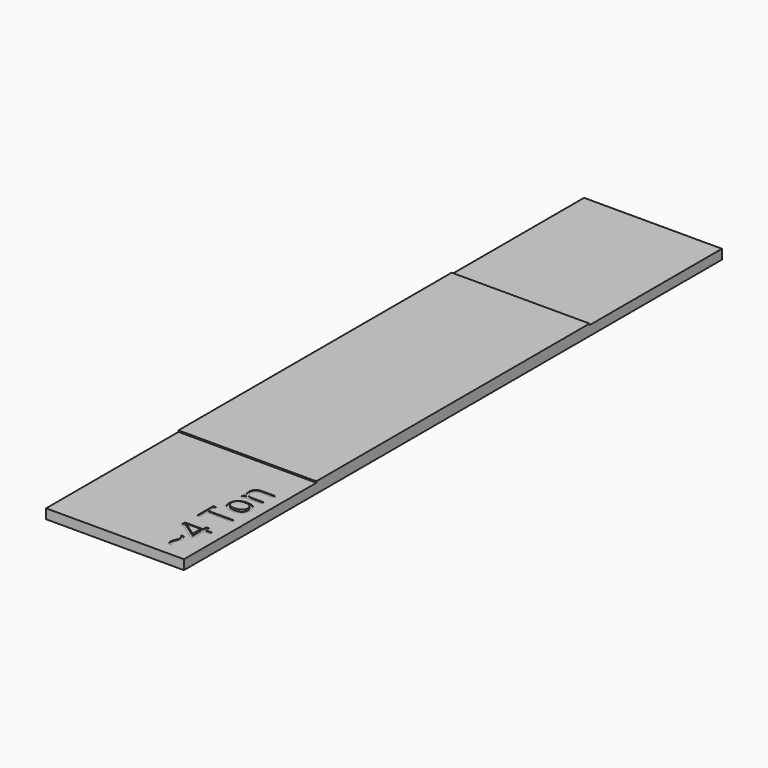
from build123d import *

# Parameters (mm, degrees)
F0_W         = 2500
F0_H         = 3000
F0_H_2       = 6192
F0_TEXT_SIZE = 689.6760728624
F1_DEPTH     = 200
F2_DEPTH     = 35
F3_DEPTH     = 25


# Not quite as in the source:
# - Text() gives the source's letters only with a copy of the font that has no kerning and outlines rounded to 1/6400 em; it was checked with that copy


with BuildPart() as f1:
    # F0 (on Top) → F1 (new body)
    with BuildSketch(Plane.XY):
        with Locations((0, -4596)):
            Rectangle(F0_W, F0_H)
        with BuildLine():
            add(Edge.make_bspline(
                [(813.513290551, -5763.3611460527), (809.4722198115, -5778.5555720329), (809.4722198115, -5794.7198549906)],
                knots=[0, 0, 0, 1, 1, 1], degree=2))
            add(Edge.make_bspline(
                [(809.4722198115, -5794.7198549906), (809.4722198115, -5812.5005662441), (820.7333369388, -5833.8913006915)],
                knots=[0, 0, 0, 1, 1, 1], degree=2))
            add(Edge.make_bspline(
                [(820.7333369388, -5833.8913006915), (831.994454066, -5855.2820351389), (850.206212865, -5873.4937939379)],
                knots=[0, 0, 0, 1, 1, 1], degree=2))
            Line((850.206212865, -5873.4937939379), (799.3426024914, -5873.4937939379))
            add(Edge.make_bspline(
                [(799.3426024914, -5873.4937939379), (762.5957992342, -5839.7643234995), (762.5957992342, -5791.2714746263)],
                knots=[0, 0, 0, 1, 1, 1], degree=2))
            add(Edge.make_bspline(
                [(762.5957992342, -5791.2714746263), (762.5957992342, -5768.4259547128), (767.3373222351, -5749.4059817659)],
                knots=[0, 0, 0, 1, 1, 1], degree=2))
            add(Edge.make_bspline(
                [(767.3373222351, -5749.4059817659), (772.078845236, -5730.3860088189), (784.9025097158, -5700.428204404)],
                knots=[0, 0, 0, 1, 1, 1], degree=2))
            add(Edge.make_bspline(
                [(784.9025097158, -5700.428204404), (794.2777938313, -5678.1214939223), (798.8576740026, -5661.6339253055)],
                knots=[0, 0, 0, 1, 1, 1], degree=2))
            add(Edge.make_bspline(
                [(798.8576740026, -5661.6339253055), (803.437554174, -5645.1463566886), (803.437554174, -5629.30535939)],
                knots=[0, 0, 0, 1, 1, 1], degree=2))
            add(Edge.make_bspline(
                [(803.437554174, -5629.30535939), (803.437554174, -5611.2013624774), (792.6613655355, -5589.6489852005)],
                knots=[0, 0, 0, 1, 1, 1], degree=2))
            add(Edge.make_bspline(
                [(792.6613655355, -5589.6489852005), (781.885176897, -5568.0966079235), (762.5957992342, -5549.8848491245)],
                knots=[0, 0, 0, 1, 1, 1], degree=2))
            Line((762.5957992342, -5549.8848491245), (813.1361239486, -5549.8848491245))
            add(Edge.make_bspline(
                [(813.1361239486, -5549.8848491245), (850.206212865, -5584.2608908812), (850.206212865, -5631.9994065497)],
                knots=[0, 0, 0, 1, 1, 1], degree=2))
            add(Edge.make_bspline(
                [(850.206212865, -5631.9994065497), (850.206212865, -5656.2458309862), (844.6564757162, -5677.474922604)],
                knots=[0, 0, 0, 1, 1, 1], degree=2))
            add(Edge.make_bspline(
                [(844.6564757162, -5677.474922604), (839.1067385674, -5698.7040142218), (828.3305499289, -5722.9504386584)],
                knots=[0, 0, 0, 1, 1, 1], degree=2))
            add(Edge.make_bspline(
                [(828.3305499289, -5722.9504386584), (817.5543612904, -5748.1667200724), (813.513290551, -5763.3611460527)],
                knots=[0, 0, 0, 1, 1, 1], degree=2))
        make_face(mode=Mode.SUBTRACT)
        Polygon((885.5521115992, -5133.7084439066), (936.4157219728, -5133.7084439066), (936.4157219728, -5206.7710028754), (1049.5657026768, -5206.7710028754), (1049.5657026768, -5260.3286604087), (936.4157219728, -5260.3286604087), (936.4157219728, -5499.7755719556), (887.5995874405, -5499.7755719556), (554.5075966252, -5266.040040387), (554.5075966252, -5206.7710028754), (885.5521115992, -5206.7710028754), align=None, mode=Mode.SUBTRACT)
        Polygon((608.0652541584, -4721.5192284849), (1049.5657026768, -4721.5192284849), (1049.5657026768, -4778.7407901552), (608.0652541584, -4778.7407901552), (608.0652541584, -4934.6722397539), (557.2016437848, -4934.6722397539), (557.2016437848, -4565.5877788862), (608.0652541584, -4565.5877788862), align=None, mode=Mode.SUBTRACT)
        with BuildLine():
            add(Edge.make_bspline(
                [(725.2563056019, -4226.9460509221), (776.820368237, -4181.3088920381), (864.6463056405, -4181.3088920381)],
                knots=[0, 0, 0, 1, 1, 1], degree=2))
            add(Edge.make_bspline(
                [(864.6463056405, -4181.3088920381), (954.950766431, -4181.3088920381), (1005.652733975, -4226.7305271493)],
                knots=[0, 0, 0, 1, 1, 1], degree=2))
            add(Edge.make_bspline(
                [(1005.652733975, -4226.7305271493), (1056.354701519, -4272.1521622605), (1056.354701519, -4352.3270057307)],
                knots=[0, 0, 0, 1, 1, 1], degree=2))
            add(Edge.make_bspline(
                [(1056.354701519, -4352.3270057307), (1056.354701519, -4401.8974734677), (1033.0781340599, -4440.2607050207)],
                knots=[0, 0, 0, 1, 1, 1], degree=2))
            add(Edge.make_bspline(
                [(1033.0781340599, -4440.2607050207), (1009.8015666008, -4478.6239365737), (966.3735263877, -4499.5297425323)],
                knots=[0, 0, 0, 1, 1, 1], degree=2))
            add(Edge.make_bspline(
                [(966.3735263877, -4499.5297425323), (922.9454861747, -4520.4355484909), (864.6463056405, -4520.4355484909)],
                knots=[0, 0, 0, 1, 1, 1], degree=2))
            add(Edge.make_bspline(
                [(864.6463056405, -4520.4355484909), (774.4496067365, -4520.4355484909), (724.0709248516, -4475.2833180957)],
                knots=[0, 0, 0, 1, 1, 1], degree=2))
            add(Edge.make_bspline(
                [(724.0709248516, -4475.2833180957), (673.6922429668, -4430.1310877005), (673.6922429668, -4349.9562442303)],
                knots=[0, 0, 0, 1, 1, 1], degree=2))
            add(Edge.make_bspline(
                [(673.6922429668, -4349.9562442303), (673.6922429668, -4272.583209806), (725.2563056019, -4226.9460509221)],
                knots=[0, 0, 0, 1, 1, 1], degree=2))
        make_face(mode=Mode.SUBTRACT)
        with BuildLine():
            Line((1049.5657026768, -3774.7232947085), (1049.5657026768, -3830.6517137421))
            Line((1049.5657026768, -3830.6517137421), (810.7653624482, -3830.6517137421))
            add(Edge.make_bspline(
                [(810.7653624482, -3830.6517137421), (765.7208939393, -3830.6517137421), (743.4680644009, -3851.1803530984)],
                knots=[0, 0, 0, 1, 1, 1], degree=2))
            add(Edge.make_bspline(
                [(743.4680644009, -3851.1803530984), (721.2152348624, -3871.7089924547), (721.2152348624, -3915.5680802133)],
                knots=[0, 0, 0, 1, 1, 1], degree=2))
            add(Edge.make_bspline(
                [(721.2152348624, -3915.5680802133), (721.2152348624, -3973.4362132019), (752.5200628572, -4000.3766847981)],
                knots=[0, 0, 0, 1, 1, 1], degree=2))
            add(Edge.make_bspline(
                [(752.5200628572, -4000.3766847981), (783.824890852, -4027.3171563943), (855.9175928434, -4027.3171563943)],
                knots=[0, 0, 0, 1, 1, 1], degree=2))
            Line((855.9175928434, -4027.3171563943), (1049.5657026768, -4027.3171563943))
            Line((1049.5657026768, -4027.3171563943), (1049.5657026768, -4083.245575428))
            Line((1049.5657026768, -4083.245575428), (680.481241809, -4083.245575428))
            Line((680.481241809, -4083.245575428), (680.481241809, -4037.7700593736))
            Line((680.481241809, -4037.7700593736), (731.0215665234, -4028.7180609173))
            Line((731.0215665234, -4028.7180609173), (731.0215665234, -4026.0240137577))
            add(Edge.make_bspline(
                [(731.0215665234, -4026.0240137577), (703.7578092681, -4008.7821119361), (688.7250261174, -3977.8005696005)],
                knots=[0, 0, 0, 1, 1, 1], degree=2))
            add(Edge.make_bspline(
                [(688.7250261174, -3977.8005696005), (673.6922429668, -3946.8190272649), (673.6922429668, -3908.7790813711)],
                knots=[0, 0, 0, 1, 1, 1], degree=2))
            add(Edge.make_bspline(
                [(673.6922429668, -3908.7790813711), (673.6922429668, -3842.0744736989), (705.8591660526, -3808.3988842037)],
                knots=[0, 0, 0, 1, 1, 1], degree=2))
            add(Edge.make_bspline(
                [(705.8591660526, -3808.3988842037), (738.0260891385, -3774.7232947085), (808.8256484932, -3774.7232947085)],
                knots=[0, 0, 0, 1, 1, 1], degree=2))
            Line((808.8256484932, -3774.7232947085), (1049.5657026768, -3774.7232947085))
        make_face(mode=Mode.SUBTRACT)
        Rectangle(F0_W, F0_H_2)
        with Locations((0, 4596)):
            Rectangle(F0_W, F0_H)
        with BuildLine():
            Line((885.5521115992, -5443.8471529219), (885.5521115992, -5260.3286604087))
            Line((885.5521115992, -5260.3286604087), (721.8618061807, -5260.3286604087))
            add(Edge.make_bspline(
                [(721.8618061807, -5260.3286604087), (673.6922429668, -5260.3286604087), (613.1300628185, -5256.8802800443)],
                knots=[0, 0, 0, 1, 1, 1], degree=2))
            Line((613.1300628185, -5256.8802800443), (613.1300628185, -5259.574327204))
            add(Edge.make_bspline(
                [(613.1300628185, -5259.574327204), (645.458628734, -5275.7386101617), (666.6877203517, -5289.9631791645)],
                knots=[0, 0, 0, 1, 1, 1], degree=2))
            Line((666.6877203517, -5289.9631791645), (885.5521115992, -5443.8471529219))
        make_face()
        with BuildLine():
            add(Edge.make_bspline(
                [(757.2615858581, -4434.4954440991), (793.3079368538, -4462.4596536159), (864.6463056405, -4462.4596536159)],
                knots=[0, 0, 0, 1, 1, 1], degree=2))
            add(Edge.make_bspline(
                [(864.6463056405, -4462.4596536159), (935.4458649953, -4462.4596536159), (972.4620729685, -4434.17215844)],
                knots=[0, 0, 0, 1, 1, 1], degree=2))
            add(Edge.make_bspline(
                [(972.4620729685, -4434.17215844), (1009.4782809416, -4405.884663264), (1009.4782809416, -4351.0338630941)],
                knots=[0, 0, 0, 1, 1, 1], degree=2))
            add(Edge.make_bspline(
                [(1009.4782809416, -4351.0338630941), (1009.4782809416, -4296.0753010379), (972.6237157981, -4267.6261630323)],
                knots=[0, 0, 0, 1, 1, 1], degree=2))
            add(Edge.make_bspline(
                [(972.6237157981, -4267.6261630323), (935.7691506545, -4239.1770250267), (864.6463056405, -4239.1770250267)],
                knots=[0, 0, 0, 1, 1, 1], degree=2))
            add(Edge.make_bspline(
                [(864.6463056405, -4239.1770250267), (794.2777938313, -4239.1770250267), (757.7465143469, -4267.6261630323)],
                knots=[0, 0, 0, 1, 1, 1], degree=2))
            add(Edge.make_bspline(
                [(757.7465143469, -4267.6261630323), (721.2152348624, -4296.0753010379), (721.2152348624, -4351.6804344124)],
                knots=[0, 0, 0, 1, 1, 1], degree=2))
            add(Edge.make_bspline(
                [(721.2152348624, -4351.6804344124), (721.2152348624, -4406.5312345823), (757.2615858581, -4434.4954440991)],
                knots=[0, 0, 0, 1, 1, 1], degree=2))
        make_face()
        with Locations(Location((1049.5657026768, -5908.5164070129), (0, 0, 90))):
            Text('~4 Ton', F0_TEXT_SIZE, font='Open Sans', text_align=(TextAlign.LEFT, TextAlign.BOTTOM))
    extrude(amount=-F1_DEPTH)

    # F0 (on Top) → F2 (cut)
    with BuildSketch(Plane.XY):
        with Locations(Location((1049.5657026768, -5908.5164070129), (0, 0, 90))):
            Text('~4 Ton', F0_TEXT_SIZE, font='Open Sans', text_align=(TextAlign.LEFT, TextAlign.BOTTOM))
    extrude(amount=-F2_DEPTH, mode=Mode.SUBTRACT)

    # F0 (on Top) → F3 (cut)
    with BuildSketch(Plane.XY):
        with Locations((0, -4596)):
            Rectangle(F0_W, F0_H)
        with BuildLine():
            add(Edge.make_bspline(
                [(813.513290551, -5763.3611460527), (809.4722198115, -5778.5555720329), (809.4722198115, -5794.7198549906)],
                knots=[0, 0, 0, 1, 1, 1], degree=2))
            add(Edge.make_bspline(
                [(809.4722198115, -5794.7198549906), (809.4722198115, -5812.5005662441), (820.7333369388, -5833.8913006915)],
                knots=[0, 0, 0, 1, 1, 1], degree=2))
            add(Edge.make_bspline(
                [(820.7333369388, -5833.8913006915), (831.994454066, -5855.2820351389), (850.206212865, -5873.4937939379)],
                knots=[0, 0, 0, 1, 1, 1], degree=2))
            Line((850.206212865, -5873.4937939379), (799.3426024914, -5873.4937939379))
            add(Edge.make_bspline(
                [(799.3426024914, -5873.4937939379), (762.5957992342, -5839.7643234995), (762.5957992342, -5791.2714746263)],
                knots=[0, 0, 0, 1, 1, 1], degree=2))
            add(Edge.make_bspline(
                [(762.5957992342, -5791.2714746263), (762.5957992342, -5768.4259547128), (767.3373222351, -5749.4059817659)],
                knots=[0, 0, 0, 1, 1, 1], degree=2))
            add(Edge.make_bspline(
                [(767.3373222351, -5749.4059817659), (772.078845236, -5730.3860088189), (784.9025097158, -5700.428204404)],
                knots=[0, 0, 0, 1, 1, 1], degree=2))
            add(Edge.make_bspline(
                [(784.9025097158, -5700.428204404), (794.2777938313, -5678.1214939223), (798.8576740026, -5661.6339253055)],
                knots=[0, 0, 0, 1, 1, 1], degree=2))
            add(Edge.make_bspline(
                [(798.8576740026, -5661.6339253055), (803.437554174, -5645.1463566886), (803.437554174, -5629.30535939)],
                knots=[0, 0, 0, 1, 1, 1], degree=2))
            add(Edge.make_bspline(
                [(803.437554174, -5629.30535939), (803.437554174, -5611.2013624774), (792.6613655355, -5589.6489852005)],
                knots=[0, 0, 0, 1, 1, 1], degree=2))
            add(Edge.make_bspline(
                [(792.6613655355, -5589.6489852005), (781.885176897, -5568.0966079235), (762.5957992342, -5549.8848491245)],
                knots=[0, 0, 0, 1, 1, 1], degree=2))
            Line((762.5957992342, -5549.8848491245), (813.1361239486, -5549.8848491245))
            add(Edge.make_bspline(
                [(813.1361239486, -5549.8848491245), (850.206212865, -5584.2608908812), (850.206212865, -5631.9994065497)],
                knots=[0, 0, 0, 1, 1, 1], degree=2))
            add(Edge.make_bspline(
                [(850.206212865, -5631.9994065497), (850.206212865, -5656.2458309862), (844.6564757162, -5677.474922604)],
                knots=[0, 0, 0, 1, 1, 1], degree=2))
            add(Edge.make_bspline(
                [(844.6564757162, -5677.474922604), (839.1067385674, -5698.7040142218), (828.3305499289, -5722.9504386584)],
                knots=[0, 0, 0, 1, 1, 1], degree=2))
            add(Edge.make_bspline(
                [(828.3305499289, -5722.9504386584), (817.5543612904, -5748.1667200724), (813.513290551, -5763.3611460527)],
                knots=[0, 0, 0, 1, 1, 1], degree=2))
        make_face(mode=Mode.SUBTRACT)
        Polygon((885.5521115992, -5133.7084439066), (936.4157219728, -5133.7084439066), (936.4157219728, -5206.7710028754), (1049.5657026768, -5206.7710028754), (1049.5657026768, -5260.3286604087), (936.4157219728, -5260.3286604087), (936.4157219728, -5499.7755719556), (887.5995874405, -5499.7755719556), (554.5075966252, -5266.040040387), (554.5075966252, -5206.7710028754), (885.5521115992, -5206.7710028754), align=None, mode=Mode.SUBTRACT)
        Polygon((608.0652541584, -4721.5192284849), (1049.5657026768, -4721.5192284849), (1049.5657026768, -4778.7407901552), (608.0652541584, -4778.7407901552), (608.0652541584, -4934.6722397539), (557.2016437848, -4934.6722397539), (557.2016437848, -4565.5877788862), (608.0652541584, -4565.5877788862), align=None, mode=Mode.SUBTRACT)
        with BuildLine():
            add(Edge.make_bspline(
                [(725.2563056019, -4226.9460509221), (776.820368237, -4181.3088920381), (864.6463056405, -4181.3088920381)],
                knots=[0, 0, 0, 1, 1, 1], degree=2))
            add(Edge.make_bspline(
                [(864.6463056405, -4181.3088920381), (954.950766431, -4181.3088920381), (1005.652733975, -4226.7305271493)],
                knots=[0, 0, 0, 1, 1, 1], degree=2))
            add(Edge.make_bspline(
                [(1005.652733975, -4226.7305271493), (1056.354701519, -4272.1521622605), (1056.354701519, -4352.3270057307)],
                knots=[0, 0, 0, 1, 1, 1], degree=2))
            add(Edge.make_bspline(
                [(1056.354701519, -4352.3270057307), (1056.354701519, -4401.8974734677), (1033.0781340599, -4440.2607050207)],
                knots=[0, 0, 0, 1, 1, 1], degree=2))
            add(Edge.make_bspline(
                [(1033.0781340599, -4440.2607050207), (1009.8015666008, -4478.6239365737), (966.3735263877, -4499.5297425323)],
                knots=[0, 0, 0, 1, 1, 1], degree=2))
            add(Edge.make_bspline(
                [(966.3735263877, -4499.5297425323), (922.9454861747, -4520.4355484909), (864.6463056405, -4520.4355484909)],
                knots=[0, 0, 0, 1, 1, 1], degree=2))
            add(Edge.make_bspline(
                [(864.6463056405, -4520.4355484909), (774.4496067365, -4520.4355484909), (724.0709248516, -4475.2833180957)],
                knots=[0, 0, 0, 1, 1, 1], degree=2))
            add(Edge.make_bspline(
                [(724.0709248516, -4475.2833180957), (673.6922429668, -4430.1310877005), (673.6922429668, -4349.9562442303)],
                knots=[0, 0, 0, 1, 1, 1], degree=2))
            add(Edge.make_bspline(
                [(673.6922429668, -4349.9562442303), (673.6922429668, -4272.583209806), (725.2563056019, -4226.9460509221)],
                knots=[0, 0, 0, 1, 1, 1], degree=2))
        make_face(mode=Mode.SUBTRACT)
        with BuildLine():
            Line((1049.5657026768, -3774.7232947085), (1049.5657026768, -3830.6517137421))
            Line((1049.5657026768, -3830.6517137421), (810.7653624482, -3830.6517137421))
            add(Edge.make_bspline(
                [(810.7653624482, -3830.6517137421), (765.7208939393, -3830.6517137421), (743.4680644009, -3851.1803530984)],
                knots=[0, 0, 0, 1, 1, 1], degree=2))
            add(Edge.make_bspline(
                [(743.4680644009, -3851.1803530984), (721.2152348624, -3871.7089924547), (721.2152348624, -3915.5680802133)],
                knots=[0, 0, 0, 1, 1, 1], degree=2))
            add(Edge.make_bspline(
                [(721.2152348624, -3915.5680802133), (721.2152348624, -3973.4362132019), (752.5200628572, -4000.3766847981)],
                knots=[0, 0, 0, 1, 1, 1], degree=2))
            add(Edge.make_bspline(
                [(752.5200628572, -4000.3766847981), (783.824890852, -4027.3171563943), (855.9175928434, -4027.3171563943)],
                knots=[0, 0, 0, 1, 1, 1], degree=2))
            Line((855.9175928434, -4027.3171563943), (1049.5657026768, -4027.3171563943))
            Line((1049.5657026768, -4027.3171563943), (1049.5657026768, -4083.245575428))
            Line((1049.5657026768, -4083.245575428), (680.481241809, -4083.245575428))
            Line((680.481241809, -4083.245575428), (680.481241809, -4037.7700593736))
            Line((680.481241809, -4037.7700593736), (731.0215665234, -4028.7180609173))
            Line((731.0215665234, -4028.7180609173), (731.0215665234, -4026.0240137577))
            add(Edge.make_bspline(
                [(731.0215665234, -4026.0240137577), (703.7578092681, -4008.7821119361), (688.7250261174, -3977.8005696005)],
                knots=[0, 0, 0, 1, 1, 1], degree=2))
            add(Edge.make_bspline(
                [(688.7250261174, -3977.8005696005), (673.6922429668, -3946.8190272649), (673.6922429668, -3908.7790813711)],
                knots=[0, 0, 0, 1, 1, 1], degree=2))
            add(Edge.make_bspline(
                [(673.6922429668, -3908.7790813711), (673.6922429668, -3842.0744736989), (705.8591660526, -3808.3988842037)],
                knots=[0, 0, 0, 1, 1, 1], degree=2))
            add(Edge.make_bspline(
                [(705.8591660526, -3808.3988842037), (738.0260891385, -3774.7232947085), (808.8256484932, -3774.7232947085)],
                knots=[0, 0, 0, 1, 1, 1], degree=2))
            Line((808.8256484932, -3774.7232947085), (1049.5657026768, -3774.7232947085))
        make_face(mode=Mode.SUBTRACT)
        with Locations((0, 4596)):
            Rectangle(F0_W, F0_H)
    extrude(amount=-F3_DEPTH, mode=Mode.SUBTRACT)


solid = f1.part
